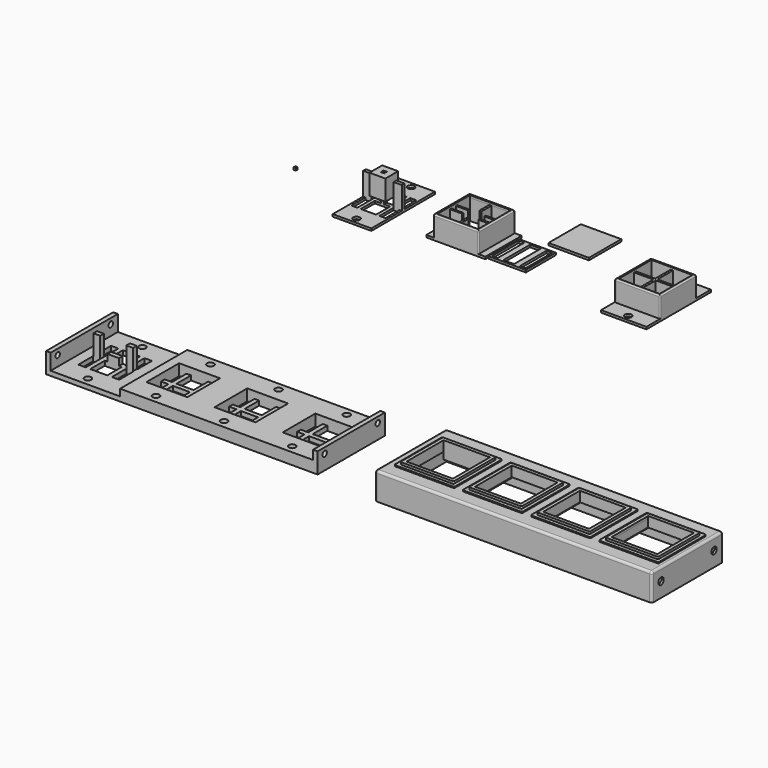
from build123d import *

# Parameters (mm, degrees)
F0_W          = 20
F0_H          = 20
F1_DEPTH      = 10
F2_T          = -1
F4_DEPTH      = 9
F5_W          = 20
F5_H          = 8
F5_R          = 1.5
F6_DEPTH      = 1
F7_W          = 20
F7_H          = 20
F8_DEPTH      = 10
F9_W          = 3
F9_H          = 20
F9_W_2        = 20
F10_DEPTH     = 0.95
F11_T         = 1
F11_T3_DEPTH  = 22
F12_W         = 8.5
F12_H         = 0.8
F13_DEPTH     = 9
F15_DEPTH     = 9
F16_W         = 17
F16_H         = 8
F16_R         = 1.5
F16_H_2       = 19
F17_DEPTH     = 1
F18_W         = 1.5
F18_H         = 1.5
F19_DEPTH     = 3
F20_W         = 7
F20_H         = 7
F20_W_2       = 1.5
F20_H_2       = 1.5
F21_DEPTH     = 9
F22_W         = 1
F22_H         = 1
F23_DEPTH     = 1
F25_DEPTH     = 10
F26_W         = 0.9
F26_H         = 14.7
F26_W_2       = 2.5
F26_H_2       = 0.8
F26_H_3       = 6
F26_H_4       = 1.1
F27_DEPTH     = 1
F28_W         = 117
F28_H         = 37
F28_R         = 1.5
F29_DEPTH     = 1
F30_W         = 122
F30_H         = 39.2
F30_W_2       = 20.4
F30_H_2       = 20.4
F30_W_3       = 20.2
F30_H_3       = 20.2
F31_DEPTH     = 11
F32_W         = 120
F32_H         = 37.2
F33_DEPTH     = 8
F34_W         = 4
F34_H         = 18
F35_DEPTH     = 3
F37_W         = 3
F37_H         = 2
F38_DEPTH     = 9
F39_W         = 5
F39_H         = 2
F40_DEPTH     = 3
F41_R         = 1
F42_R         = 0.5
F42_2_R       = 0.5
F36_R         = 1.5
F43_DEPTH     = 3
F44_DEPTH     = 2
F45_W         = 2
F45_H         = 37
F46_DEPTH     = 7
F47_W         = 20.4
F47_H         = 8.4
F48_DEPTH     = 3
F49_R         = 1.5
F50_DEPTH     = 3
F52_R         = 1.5
F53_DEPTH     = 2
F54_W         = 3
F54_H         = 37.2
F55_DEPTH     = 1
F56_DEPTH     = 1
F57_W         = 2
F57_H         = 37
F58_DEPTH     = 4
F51_R         = 1.2
F59_DEPTH     = 269.2358512024
F60_DEPTH     = 3
F61_DEPTH     = 5
F44_FACE2_W   = 119
F44_FACE2_H   = 37
F44_FACE2_R   = 1.5
F44_FACE2_W_2 = 3.25
F44_FACE2_H_2 = 8
F44_FACE2_W_3 = 7.5
F62_DEPTH     = 1
F63_DEPTH     = 1
F64_DEPTH     = 2
F65_DEPTH     = 0.05
F66_W         = 20.4
F66_H         = 3
F66_W_2       = 20.2
F66_H_2       = 3.1
F67_DEPTH     = 0.5
F68_W         = 20.4
F68_H         = 1.5
F68_W_2       = 20.2
F69_DEPTH     = 1
F70_R         = 0.5
F71_W         = 18
F71_H         = 17.9999990673
F72_DEPTH     = 1
F73_W         = 17.8
F73_H         = 17.8
F74_DEPTH     = 1
F75_W         = 18
F75_H         = 18
F76_DEPTH     = 1


# Not quite as in the source:
# - a shell that OpenCascade refuses in one call is made with other operations: the cavity is built on its own and cut out
# - a feature names something its author has since deleted; it is built from what else it names


with BuildPart() as f1:
    # F0 (on Top) → F1 (new body)
    with BuildSketch(Plane.XY):
        Rectangle(F0_W, F0_H)
    extrude(amount=F1_DEPTH)

    # F2
    f2_openings = [f1.faces().sort_by_distance(p)[0] for p in [
        (0, 0, 0),
    ]]
    offset(amount=F2_T, openings=f2_openings)

    # F3 (on Top) → F4 (join)
    with BuildSketch(Plane.XY):
        Polygon((-0.5, -9), (0.5, -9), (0.5, -0.5), (9, -0.5), (9, 0.5), (0.5, 0.5), (0.5, 9), (-0.5, 9), (-0.5, 0.5), (-9, 0.5), (-9, -0.5), (-0.5, -0.5), align=None)
    extrude(amount=F4_DEPTH)

    # F5 (on Top) → F6 (join)
    with BuildSketch(Plane.XY):
        with Locations((0, -13.5)):
            Rectangle(F5_W, F5_H)
        with Locations((0, -15)):
            Circle(F5_R, mode=Mode.SUBTRACT)
        with Locations((0, 14)):
            Rectangle(F5_W, F5_H)
        with Locations((0, 15)):
            Circle(F5_R, mode=Mode.SUBTRACT)
    extrude(amount=F6_DEPTH)

    # F42
    f42_edges = [f1.edges().sort_by_distance(p)[0] for p in [
        (-10, -10, 5.5),
        (0, -10, 10),
        (10, -10, 5.5),
        (-10, 0, 10),
        (-10, 10, 5.5),
        (0, 10, 10),
        (10, 10, 5.5),
        (10, 0, 10),
    ]]
    fillet(f42_edges, radius=F42_R)

    # F75 (on face) → F76 (cut)
    with BuildSketch(Plane.XY.offset(10)):
        Rectangle(F75_W, F75_H)
    extrude(amount=-F76_DEPTH, mode=Mode.SUBTRACT)


with BuildPart() as f8:
    # F7 (on Top) → F8 (new body)
    with BuildSketch(Plane.XY):
        with Locations((-78.8846665621, -1.3073290847)):
            Rectangle(F7_W, F7_H)
    extrude(amount=F8_DEPTH)

    # F9 (on face) → F10 (join)
    with BuildSketch(Plane(origin=(0, 0, 0), x_dir=(1, 0, 0), z_dir=(0, 0, -1))):
        with Locations((-90.3846665621, 1.3073290847)):
            Rectangle(F9_W, F9_H)
        with Locations((-78.8846665621, 1.3073290847)):
            Rectangle(F9_W_2, F9_H)
        with Locations((-67.3846665621, 1.3073290847)):
            Rectangle(F9_W, F9_H)
    extrude(amount=-F10_DEPTH)

    # F11: shell of thickness 1, made by hand


with BuildPart() as f11_core1:
    # F11_t2: copy of F8
    add(f8.part)

    # the walls: a layer under each face that stays
    f11_faces = [f11_core1.faces().sort_by_distance(p)[0] for p in [
        (-78.8846665621, 8.6926709153, 5),
        (-91.8846665621, -1.3073290847, 0.475),
        (-78.8846665621, -11.3073290847, 5),
        (-90.3846665621, -1.3073290847, 0.95),
        (-88.8846665621, -1.3073290847, 5.475),
        (-78.8846665621, -1.3073290847, 10),
        (-68.8846665621, -1.3073290847, 5.475),
        (-67.3846665621, -1.3073290847, 0.95),
        (-65.8846665621, -1.3073290847, 0.475),
    ]]
    thicken(f11_faces, amount=-F11_T, mode=Mode.SUBTRACT)

    # F11_s4 → F11_t3 (cut)
    with BuildSketch(Plane.XZ.offset(-9.6926709153)):
        Polygon((-88.8946665621, 0.96), (-88.8846665621, -0.05), (-87.8846665621, -0.05), (-87.8846665621, 0.95), align=None)
        Polygon((-68.8746665621, 0.96), (-69.8846665621, 0.95), (-69.8846665621, -0.05), (-68.8846665621, -0.05), align=None)
    extrude(amount=F11_T3_DEPTH, mode=Mode.SUBTRACT)


with BuildPart() as f8_1:
    add(f8.part)

    # what is left inside the walls is the cavity
    f11_cavity = [f11_core1.part.solids().sort_by_distance(p)[0] for p in [
        (-78.884667, -4.307329, 0.01),
    ]]
    add(f11_cavity, mode=Mode.SUBTRACT)

    # F12 (on Top) → F13 (join)
    with BuildSketch(Plane.XY):
        Polygon((-78.3846665621, 7.6926709153), (-79.3846665621, 7.6926709153), (-79.3846665621, 0.6926709153), (-79.3846665621, -0.1073290847), (-79.3846665621, -2.5073290847), (-79.3846665621, -3.3073290847), (-79.3846665621, -10.3073290847), (-78.3846665621, -10.3073290847), (-78.3846665621, -3.3073290847), (-78.3846665621, -2.5073290847), (-78.3846665621, -0.1073290847), (-78.3846665621, 0.6926709153), align=None)
        with Locations((-83.6346665621, -2.9073290847)):
            Rectangle(F12_W, F12_H)
        with Locations((-83.6346665621, 0.2926709153)):
            Rectangle(F12_W, F12_H)
        with Locations((-74.1346665621, 0.2926709153)):
            Rectangle(F12_W, F12_H)
        with Locations((-74.1346665621, -2.9073290847)):
            Rectangle(F12_W, F12_H)
    extrude(amount=F13_DEPTH)

    # F14 (on face) → F15 (cut)
    with BuildSketch(Plane(origin=(0, 0, 0), x_dir=(1, 0, 0), z_dir=(0, 0, -1))):
        Polygon((-79.3846665621, -2.2926709153), (-78.3846665621, -2.2926709153), (-78.3846665621, -0.6926709153), (-75.2846665621, -0.6926709153), (-75.2846665621, 0.1073290847), (-78.3846665621, 0.1073290847), (-78.3846665621, 2.5073290847), (-75.2846665621, 2.5073290847), (-75.2846665621, 3.3073290847), (-78.3846665621, 3.3073290847), (-78.3846665621, 4.9073290847), (-79.3846665621, 4.9073290847), (-79.3846665621, 3.3073290847), (-82.4846665621, 3.3073290847), (-82.4846665621, 2.5073290847), (-79.3846665621, 2.5073290847), (-79.3846665621, 0.1073290847), (-82.4846665621, 0.1073290847), (-82.4846665621, -0.6926709153), (-79.3846665621, -0.6926709153), align=None)
    extrude(amount=-F15_DEPTH, mode=Mode.SUBTRACT)

    # F42#2
    f42_2_edges = [f8_1.edges().sort_by_distance(p)[0] for p in [
        (-68.884667, -11.307329, 5.475),
        (-78.884667, -11.307329, 10),
        (-68.884667, -1.307329, 10),
        (-68.884667, 8.692671, 5.475),
        (-78.884667, 8.692671, 10),
        (-88.884667, 8.692671, 5.475),
        (-88.884667, -1.307329, 10),
        (-88.884667, -11.307329, 5.475),
    ]]
    fillet(f42_2_edges, radius=F42_2_R)

    # F65 (add): faces of the model
    f65_faces = [f8_1.faces().sort_by_distance(p)[0] for p in [
        (-90.3817894545, -1.3073290847, 0.95),
        (-67.3875436696, -1.3073290847, 0.95),
    ]]
    extrude(f65_faces, amount=F65_DEPTH)

    # F71 (on face) → F72 (cut)
    with BuildSketch(Plane.XY.offset(10)):
        with Locations((-78.8846665621, -1.3073295511)):
            Rectangle(F71_W, F71_H)
    extrude(amount=-F72_DEPTH, mode=Mode.SUBTRACT)


with BuildPart() as f17:
    # F16 (on Top) → F17 (new body)
    with BuildSketch(Plane.XY):
        with Locations((-118.1940851788, 11.6607970074)):
            Rectangle(F16_W, F16_H)
        with Locations((-118.1940851788, 13.1607970074)):
            Circle(F16_R, mode=Mode.SUBTRACT)
        with Locations((-118.1940851788, -15.3392029926)):
            Rectangle(F16_W, F16_H)
        with Locations((-118.1940851788, -16.8392029926)):
            Circle(F16_R, mode=Mode.SUBTRACT)
        with Locations((-118.1940851788, -1.8392029926)):
            Rectangle(F16_W, F16_H_2)
        Polygon((-125.6940851788, -1.0892029926), (-125.6940851788, 6.6607970074), (-123.0690851788, 6.6607970074), (-121.5690851788, 6.6607970074), (-114.8190851788, 6.6607970074), (-113.3190851788, 6.6607970074), (-110.6940851788, 6.6607970074), (-110.6940851788, -1.0892029926), (-110.6940851788, -2.5892029926), (-110.6940851788, -10.3392029926), (-113.3190851788, -10.3392029926), (-114.8190851788, -10.3392029926), (-121.5690851788, -10.3392029926), (-123.0690851788, -10.3392029926), (-125.6940851788, -10.3392029926), (-125.6940851788, -2.5892029926), align=None, mode=Mode.SUBTRACT)
        Polygon((-121.5690851788, 6.6607970074), (-123.0690851788, 6.6607970074), (-123.0690851788, -1.0892029926), (-125.6940851788, -1.0892029926), (-125.6940851788, -2.5892029926), (-123.0690851788, -2.5892029926), (-123.0690851788, -10.3392029926), (-121.5690851788, -10.3392029926), (-121.5690851788, -2.5892029926), (-114.8190851788, -2.5892029926), (-114.8190851788, -10.3392029926), (-113.3190851788, -10.3392029926), (-113.3190851788, -2.5892029926), (-110.6940851788, -2.5892029926), (-110.6940851788, -1.0892029926), (-113.3190851788, -1.0892029926), (-113.3190851788, 6.6607970074), (-114.8190851788, 6.6607970074), (-114.8190851788, -1.0892029926), (-121.5690851788, -1.0892029926), align=None)
    extrude(amount=F17_DEPTH)

    # F18 (on face) → F19 (join)
    with BuildSketch(Plane.XY.offset(1)):
        with Locations((-118.1940851788, -1.8392029926)):
            Rectangle(F18_W, F18_H)
    extrude(amount=F19_DEPTH)

    # F24 (on face) → F25 (join)
    with BuildSketch(Plane.XY.offset(1)):
        Polygon((-109.6940851788, -2.5892029926), (-109.6940851788, -1.0892029926), (-110.6940851788, -1.0892029926), (-113.3190851788, -1.0892029926), (-113.3190851788, -2.5892029926), (-110.6940851788, -2.5892029926), align=None)
        Polygon((-125.6940851788, -1.0892029926), (-126.6940851788, -1.0892029926), (-126.6940851788, -2.5892029926), (-125.6940851788, -2.5892029926), (-123.0690851788, -2.5892029926), (-123.0690851788, -1.0892029926), align=None)
    extrude(amount=F25_DEPTH)


with BuildPart() as f21:
    # F20 (on face) → F21 (new body)
    with BuildSketch(Plane.XY.offset(4)):
        with Locations((-118.1940851788, -1.8392029926)):
            Rectangle(F20_W, F20_H)
        with Locations((-118.1940851788, -1.8392029926)):
            Rectangle(F20_W_2, F20_H_2, mode=Mode.SUBTRACT)
    extrude(amount=F21_DEPTH)


with BuildPart() as f23:
    # F22 (on Top) → F23 (new body)
    with BuildSketch(Plane.XY):
        with Locations((-158.5527062416, 0)):
            Rectangle(F22_W, F22_H)
    extrude(amount=F23_DEPTH)


with BuildPart() as f27:
    # F26 (on Top) → F27 (new body)
    with BuildSketch(Plane.XY):
        Polygon((-64.4713718057, -9.4157041669), (-65.3713718057, -9.4157041669), (-65.3713718057, -10.3157041669), (-54.7713718057, -10.3157041669), (-52.2713718057, -10.3157041669), (-48.8713718057, -10.3157041669), (-48.8713718057, -9.4157041669), (-49.7713718057, -9.4157041669), (-52.2713718057, -9.4157041669), (-54.7713718057, -9.4157041669), (-59.4713718057, -9.4157041669), (-61.9713718057, -9.4157041669), align=None)
        with Locations((-64.9213718057, -2.0657041669)):
            Rectangle(F26_W, F26_H)
        Polygon((-48.8713718057, 6.1842958331), (-65.3713718057, 6.1842958331), (-65.3713718057, 5.2842958331), (-64.4713718057, 5.2842958331), (-61.9713718057, 5.2842958331), (-59.4713718057, 5.2842958331), (-54.7713718057, 5.2842958331), (-52.2713718057, 5.2842958331), (-49.7713718057, 5.2842958331), (-48.8713718057, 5.2842958331), align=None)
        with Locations((-49.3213718057, -2.0657041669)):
            Rectangle(F26_W, F26_H)
        with Locations((-53.5213718057, 4.8842958331)):
            Rectangle(F26_W_2, F26_H_2)
        with Locations((-53.5213718057, 1.4842958331)):
            Rectangle(F26_W_2, F26_H_3)
        with Locations((-53.5213718057, -2.0657041669)):
            Rectangle(F26_W_2, F26_H_4)
        with Locations((-53.5213718057, -5.6157041669)):
            Rectangle(F26_W_2, F26_H_3)
        with Locations((-53.5213718057, -9.0157041669)):
            Rectangle(F26_W_2, F26_H_2)
        with Locations((-60.7213718057, 4.8842958331)):
            Rectangle(F26_W_2, F26_H_2)
        with Locations((-60.7213718057, 1.4842958331)):
            Rectangle(F26_W_2, F26_H_3)
        with Locations((-60.7213718057, -2.0657041669)):
            Rectangle(F26_W_2, F26_H_4)
        with Locations((-60.7213718057, -5.6157041669)):
            Rectangle(F26_W_2, F26_H_3)
        with Locations((-60.7213718057, -9.0157041669)):
            Rectangle(F26_W_2, F26_H_2)
    extrude(amount=F27_DEPTH)


with BuildPart() as f29:
    # F28 (on Top) → F29 (new body)
    with BuildSketch(Plane.XY):
        with Locations((-71.0754835367, -152.5580135584)):
            Rectangle(F28_W, F28_H)
        with Locations((-115.9754835367, -167.5580135584)):
            Circle(F28_R, mode=Mode.SUBTRACT)
        with Locations((-85.9754835367, -167.5580135584)):
            Circle(F28_R, mode=Mode.SUBTRACT)
        Polygon((-124.9754835367, -151.5580135584), (-124.9754835367, -143.5580135584), (-121.7254835367, -143.5580135584), (-119.7254835367, -143.5580135584), (-112.2254835367, -143.5580135584), (-110.2254835367, -143.5580135584), (-106.9754835367, -143.5580135584), (-106.9754835367, -151.5580135584), (-106.9754835367, -153.5580135584), (-106.9754835367, -161.5580135584), (-110.2254835367, -161.5580135584), (-112.2254835367, -161.5580135584), (-119.7254835367, -161.5580135584), (-121.7254835367, -161.5580135584), (-124.9754835367, -161.5580135584), (-124.9754835367, -153.5580135584), align=None, mode=Mode.SUBTRACT)
        Polygon((-94.9754835367, -151.5580135584), (-94.9754835367, -143.5580135584), (-91.7254835367, -143.5580135584), (-89.7254835367, -143.5580135584), (-82.2254835367, -143.5580135584), (-80.2254835367, -143.5580135584), (-76.9754835367, -143.5580135584), (-76.9754835367, -151.5580135584), (-76.9754835367, -153.5580135584), (-76.9754835367, -161.5580135584), (-80.2254835367, -161.5580135584), (-82.2254835367, -161.5580135584), (-89.7254835367, -161.5580135584), (-91.7254835367, -161.5580135584), (-94.9754835367, -161.5580135584), (-94.9754835367, -153.5580135584), align=None, mode=Mode.SUBTRACT)
        with Locations((-55.9754835367, -167.5580135584)):
            Circle(F28_R, mode=Mode.SUBTRACT)
        with Locations((-25.9754835367, -167.5580135584)):
            Circle(F28_R, mode=Mode.SUBTRACT)
        Polygon((-64.9754835367, -151.5580135584), (-64.9754835367, -143.5580135584), (-61.7254835367, -143.5580135584), (-59.7254835367, -143.5580135584), (-52.2254835367, -143.5580135584), (-50.2254835367, -143.5580135584), (-46.9754835367, -143.5580135584), (-46.9754835367, -151.5580135584), (-46.9754835367, -153.5580135584), (-46.9754835367, -161.5580135584), (-47.9754835367, -161.5580135584), (-50.2254835367, -161.5580135584), (-52.2254835367, -161.5580135584), (-59.7254835367, -161.5580135584), (-61.7254835367, -161.5580135584), (-64.9754835367, -161.5580135584), (-64.9754835367, -153.5580135584), align=None, mode=Mode.SUBTRACT)
        Polygon((-34.9754835367, -151.5580135584), (-34.9754835367, -143.5580135584), (-31.7254835367, -143.5580135584), (-29.7254835367, -143.5580135584), (-22.2254835367, -143.5580135584), (-20.2254835367, -143.5580135584), (-16.9754835367, -143.5580135584), (-16.9754835367, -151.5580135584), (-16.9754835367, -153.5580135584), (-16.9754835367, -161.5580135584), (-17.9754835367, -161.5580135584), (-20.2254835367, -161.5580135584), (-22.2254835367, -161.5580135584), (-29.7254835367, -161.5580135584), (-31.7254835367, -161.5580135584), (-34.9754835367, -161.5580135584), (-34.9754835367, -153.5580135584), align=None, mode=Mode.SUBTRACT)
        with Locations((-115.9754835367, -137.5580135584)):
            Circle(F28_R, mode=Mode.SUBTRACT)
        with Locations((-85.9754835367, -137.5580135584)):
            Circle(F28_R, mode=Mode.SUBTRACT)
        with Locations((-55.9754835367, -137.5580135584)):
            Circle(F28_R, mode=Mode.SUBTRACT)
        with Locations((-25.9754835367, -137.5580135584)):
            Circle(F28_R, mode=Mode.SUBTRACT)
        Polygon((-119.7254835367, -143.5580135584), (-121.7254835367, -143.5580135584), (-121.7254835367, -151.5580135584), (-124.9754835367, -151.5580135584), (-124.9754835367, -153.5580135584), (-121.7254835367, -153.5580135584), (-121.7254835367, -161.5580135584), (-119.7254835367, -161.5580135584), (-119.7254835367, -153.5580135584), (-112.2254835367, -153.5580135584), (-112.2254835367, -161.5580135584), (-110.2254835367, -161.5580135584), (-110.2254835367, -153.5580135584), (-106.9754835367, -153.5580135584), (-106.9754835367, -151.5580135584), (-110.2254835367, -151.5580135584), (-110.2254835367, -143.5580135584), (-112.2254835367, -143.5580135584), (-112.2254835367, -151.5580135584), (-119.7254835367, -151.5580135584), align=None)
        Polygon((-89.7254835367, -143.5580135584), (-91.7254835367, -143.5580135584), (-91.7254835367, -151.5580135584), (-94.9754835367, -151.5580135584), (-94.9754835367, -153.5580135584), (-91.7254835367, -153.5580135584), (-91.7254835367, -161.5580135584), (-89.7254835367, -161.5580135584), (-89.7254835367, -153.5580135584), (-82.2254835367, -153.5580135584), (-82.2254835367, -161.5580135584), (-80.2254835367, -161.5580135584), (-80.2254835367, -153.5580135584), (-76.9754835367, -153.5580135584), (-76.9754835367, -151.5580135584), (-80.2254835367, -151.5580135584), (-80.2254835367, -143.5580135584), (-82.2254835367, -143.5580135584), (-82.2254835367, -151.5580135584), (-89.7254835367, -151.5580135584), align=None)
        Polygon((-59.7254835367, -143.5580135584), (-61.7254835367, -143.5580135584), (-61.7254835367, -151.5580135584), (-64.9754835367, -151.5580135584), (-64.9754835367, -153.5580135584), (-61.7254835367, -153.5580135584), (-61.7254835367, -161.5580135584), (-59.7254835367, -161.5580135584), (-59.7254835367, -153.5580135584), (-52.2254835367, -153.5580135584), (-52.2254835367, -161.5580135584), (-50.2254835367, -161.5580135584), (-50.2254835367, -153.5580135584), (-46.9754835367, -153.5580135584), (-46.9754835367, -151.5580135584), (-50.2254835367, -151.5580135584), (-50.2254835367, -143.5580135584), (-52.2254835367, -143.5580135584), (-52.2254835367, -151.5580135584), (-59.7254835367, -151.5580135584), align=None)
        Polygon((-29.7254835367, -143.5580135584), (-31.7254835367, -143.5580135584), (-31.7254835367, -151.5580135584), (-34.9754835367, -151.5580135584), (-34.9754835367, -153.5580135584), (-31.7254835367, -153.5580135584), (-31.7254835367, -161.5580135584), (-29.7254835367, -161.5580135584), (-29.7254835367, -153.5580135584), (-22.2254835367, -153.5580135584), (-22.2254835367, -161.5580135584), (-20.2254835367, -161.5580135584), (-20.2254835367, -153.5580135584), (-16.9754835367, -153.5580135584), (-16.9754835367, -151.5580135584), (-20.2254835367, -151.5580135584), (-20.2254835367, -143.5580135584), (-22.2254835367, -143.5580135584), (-22.2254835367, -151.5580135584), (-29.7254835367, -151.5580135584), align=None)
    extrude(amount=F29_DEPTH)

    # F34 (on face) → F35 (join)
    with BuildSketch(Plane.XY.offset(1)):
        with Locations((-96.9754835367, -152.5580135584)):
            Rectangle(F34_W, F34_H)
        with Locations((-74.9754835367, -152.5580135584)):
            Rectangle(F34_W, F34_H)
        with Locations((-66.9754835367, -152.5580135584)):
            Rectangle(F34_W, F34_H)
        with Locations((-44.9754835367, -152.5580135584)):
            Rectangle(F34_W, F34_H)
        with Locations((-36.9754835367, -152.5580135584)):
            Rectangle(F34_W, F34_H)
        with Locations((-14.9754835367, -152.5580135584)):
            Rectangle(F34_W, F34_H)
    extrude(amount=F35_DEPTH)

    # F37 (on face) → F38 (join)
    with BuildSketch(Plane.XY.offset(1)):
        with Locations((-123.2254835367, -152.5580135584)):
            Rectangle(F37_W, F37_H)
        with Locations((-108.7254835367, -152.5580135584)):
            Rectangle(F37_W, F37_H)
    extrude(amount=F38_DEPTH)

    # F39 (on face) → F40 (join)
    with BuildSketch(Plane.XY.offset(1)):
        with Locations((-115.9754835367, -152.5580135584)):
            Rectangle(F39_W, F39_H)
    extrude(amount=F40_DEPTH)

    # F36 (on face) → F43 (join)
    with BuildSketch(Plane.XY.offset(1)):
        Polygon((-98.9754835367, -134.0580135584), (-98.9754835367, -143.5580135584), (-94.9754835367, -143.5580135584), (-91.7254835367, -143.5580135584), (-89.7254835367, -143.5580135584), (-82.2254835367, -143.5580135584), (-80.2254835367, -143.5580135584), (-76.9754835367, -143.5580135584), (-72.9754835367, -143.5580135584), (-72.9754835367, -134.0580135584), align=None)
        with Locations((-85.9754835367, -137.5580135584)):
            Circle(F36_R, mode=Mode.SUBTRACT)
        Polygon((-94.9754835367, -161.5580135584), (-98.9754835367, -161.5580135584), (-98.9754835367, -171.0580135584), (-72.9754835367, -171.0580135584), (-72.9754835367, -161.5580135584), (-76.9754835367, -161.5580135584), (-80.2254835367, -161.5580135584), (-82.2254835367, -161.5580135584), (-89.7254835367, -161.5580135584), (-91.7254835367, -161.5580135584), align=None)
        with Locations((-85.9754835367, -167.5580135584)):
            Circle(F36_R, mode=Mode.SUBTRACT)
        Polygon((-68.9754835367, -161.5580135584), (-68.9754835367, -171.0580135584), (-42.9754835367, -171.0580135584), (-42.9754835367, -161.5580135584), (-46.9754835367, -161.5580135584), (-50.2254835367, -161.5580135584), (-52.2254835367, -161.5580135584), (-59.7254835367, -161.5580135584), (-61.7254835367, -161.5580135584), (-64.9754835367, -161.5580135584), align=None)
        with Locations((-55.9754835367, -167.5580135584)):
            Circle(F36_R, mode=Mode.SUBTRACT)
        Polygon((-42.9754835367, -134.0580135584), (-68.9754835367, -134.0580135584), (-68.9754835367, -143.5580135584), (-64.9754835367, -143.5580135584), (-61.7254835367, -143.5580135584), (-59.7254835367, -143.5580135584), (-52.2254835367, -143.5580135584), (-50.2254835367, -143.5580135584), (-46.9754835367, -143.5580135584), (-42.9754835367, -143.5580135584), align=None)
        with Locations((-55.9754835367, -137.5580135584)):
            Circle(F36_R, mode=Mode.SUBTRACT)
        Polygon((-12.9754835367, -134.0580135584), (-38.9754835367, -134.0580135584), (-38.9754835367, -143.5580135584), (-34.9754835367, -143.5580135584), (-31.7254835367, -143.5580135584), (-29.7254835367, -143.5580135584), (-22.2254835367, -143.5580135584), (-20.2254835367, -143.5580135584), (-16.9754835367, -143.5580135584), (-12.9754835367, -143.5580135584), align=None)
        with Locations((-25.9754835367, -137.5580135584)):
            Circle(F36_R, mode=Mode.SUBTRACT)
        Polygon((-38.9754835367, -161.5580135584), (-38.9754835367, -171.0580135584), (-12.9754835367, -171.0580135584), (-12.9754835367, -161.5580135584), (-16.9754835367, -161.5580135584), (-20.2254835367, -161.5580135584), (-22.2254835367, -161.5580135584), (-29.7254835367, -161.5580135584), (-31.7254835367, -161.5580135584), (-34.9754835367, -161.5580135584), align=None)
        with Locations((-25.9754835367, -167.5580135584)):
            Circle(F36_R, mode=Mode.SUBTRACT)
    extrude(amount=F43_DEPTH)

    # F44 (add): a face of the model
    f44_faces = [f29.faces().sort_by_distance(p)[0] for p in [
        (-129.5754835367, -152.5580135584, 0.5),
    ]]
    extrude(f44_faces, amount=F44_DEPTH)

    # F45 (on face) → F46 (join)
    with BuildSketch(Plane.XY.offset(1)):
        with Locations((-130.5754835367, -152.5580135584)):
            Rectangle(F45_W, F45_H)
    extrude(amount=F46_DEPTH)

    # F56 (add): a face of the model
    f56_faces = [f29.faces().sort_by_distance(p)[0] for p in [
        (-12.9754835367, -152.5580135584, 2.5),
    ]]
    extrude(f56_faces, amount=F56_DEPTH)

    # F57 (on face) → F58 (join)
    with BuildSketch(Plane.XY.offset(4)):
        with Locations((-12.9754835367, -152.5580135584)):
            Rectangle(F57_W, F57_H)
    extrude(amount=F58_DEPTH)

    # F51 (on face) → F59 (cut, through all)
    with BuildSketch(Plane(origin=(-131.5754835367, 0, 0), x_dir=(0, -1, 0), z_dir=(-1, 0, 0))):
        with Locations((137.9580135584, 5.5)):
            Circle(F51_R)
        with Locations((167.1580135584, 5.5)):
            Circle(F51_R)
    extrude(amount=-F59_DEPTH, mode=Mode.SUBTRACT)

    # F61 (add): faces of the model
    f61_faces = [f29.faces().sort_by_distance(p)[0] for p in [
        (-72.9754835367, -152.5580135584, 2.5),
        (-42.9754835367, -152.5580135584, 2.5),
    ]]
    extrude(f61_faces, amount=F61_DEPTH)

    # F28 (on Top) + F44_face2 (on face) → F62 (join)
    with BuildSketch(Plane.XY):
        with Locations((-71.0754835367, -152.5580135584)):
            Rectangle(F28_W, F28_H)
        with Locations((-115.9754835367, -167.5580135584)):
            Circle(F28_R, mode=Mode.SUBTRACT)
        with Locations((-85.9754835367, -167.5580135584)):
            Circle(F28_R, mode=Mode.SUBTRACT)
        Polygon((-124.9754835367, -151.5580135584), (-124.9754835367, -143.5580135584), (-121.7254835367, -143.5580135584), (-119.7254835367, -143.5580135584), (-112.2254835367, -143.5580135584), (-110.2254835367, -143.5580135584), (-106.9754835367, -143.5580135584), (-106.9754835367, -151.5580135584), (-106.9754835367, -153.5580135584), (-106.9754835367, -161.5580135584), (-110.2254835367, -161.5580135584), (-112.2254835367, -161.5580135584), (-119.7254835367, -161.5580135584), (-121.7254835367, -161.5580135584), (-124.9754835367, -161.5580135584), (-124.9754835367, -153.5580135584), align=None, mode=Mode.SUBTRACT)
        Polygon((-94.9754835367, -151.5580135584), (-94.9754835367, -143.5580135584), (-91.7254835367, -143.5580135584), (-89.7254835367, -143.5580135584), (-82.2254835367, -143.5580135584), (-80.2254835367, -143.5580135584), (-76.9754835367, -143.5580135584), (-76.9754835367, -151.5580135584), (-76.9754835367, -153.5580135584), (-76.9754835367, -161.5580135584), (-80.2254835367, -161.5580135584), (-82.2254835367, -161.5580135584), (-89.7254835367, -161.5580135584), (-91.7254835367, -161.5580135584), (-94.9754835367, -161.5580135584), (-94.9754835367, -153.5580135584), align=None, mode=Mode.SUBTRACT)
        with Locations((-55.9754835367, -167.5580135584)):
            Circle(F28_R, mode=Mode.SUBTRACT)
        with Locations((-25.9754835367, -167.5580135584)):
            Circle(F28_R, mode=Mode.SUBTRACT)
        Polygon((-64.9754835367, -151.5580135584), (-64.9754835367, -143.5580135584), (-61.7254835367, -143.5580135584), (-59.7254835367, -143.5580135584), (-52.2254835367, -143.5580135584), (-50.2254835367, -143.5580135584), (-46.9754835367, -143.5580135584), (-46.9754835367, -151.5580135584), (-46.9754835367, -153.5580135584), (-46.9754835367, -161.5580135584), (-47.9754835367, -161.5580135584), (-50.2254835367, -161.5580135584), (-52.2254835367, -161.5580135584), (-59.7254835367, -161.5580135584), (-61.7254835367, -161.5580135584), (-64.9754835367, -161.5580135584), (-64.9754835367, -153.5580135584), align=None, mode=Mode.SUBTRACT)
        Polygon((-34.9754835367, -151.5580135584), (-34.9754835367, -143.5580135584), (-31.7254835367, -143.5580135584), (-29.7254835367, -143.5580135584), (-22.2254835367, -143.5580135584), (-20.2254835367, -143.5580135584), (-16.9754835367, -143.5580135584), (-16.9754835367, -151.5580135584), (-16.9754835367, -153.5580135584), (-16.9754835367, -161.5580135584), (-17.9754835367, -161.5580135584), (-20.2254835367, -161.5580135584), (-22.2254835367, -161.5580135584), (-29.7254835367, -161.5580135584), (-31.7254835367, -161.5580135584), (-34.9754835367, -161.5580135584), (-34.9754835367, -153.5580135584), align=None, mode=Mode.SUBTRACT)
        with Locations((-115.9754835367, -137.5580135584)):
            Circle(F28_R, mode=Mode.SUBTRACT)
        with Locations((-85.9754835367, -137.5580135584)):
            Circle(F28_R, mode=Mode.SUBTRACT)
        with Locations((-55.9754835367, -137.5580135584)):
            Circle(F28_R, mode=Mode.SUBTRACT)
        with Locations((-25.9754835367, -137.5580135584)):
            Circle(F28_R, mode=Mode.SUBTRACT)
    with BuildSketch(Plane(origin=(-72.3791549796, -152.5580135584, 0), x_dir=(1, 0, 0), z_dir=(0, 0, -1))):
        with Locations((0.3036714428, 0)):
            Rectangle(F44_FACE2_W, F44_FACE2_H)
        with Locations((-43.5963285572, 15)):
            Circle(F44_FACE2_R, mode=Mode.SUBTRACT)
        with Locations((-13.5963285572, 15)):
            Circle(F44_FACE2_R, mode=Mode.SUBTRACT)
        with Locations((-36.2213285572, 5)):
            Rectangle(F44_FACE2_W_2, F44_FACE2_H_2, mode=Mode.SUBTRACT)
        with Locations((-43.5963285572, 5)):
            Rectangle(F44_FACE2_W_3, F44_FACE2_H_2, mode=Mode.SUBTRACT)
        with Locations((-50.9713285572, 5)):
            Rectangle(F44_FACE2_W_2, F44_FACE2_H_2, mode=Mode.SUBTRACT)
        with Locations((-50.9713285572, -5)):
            Rectangle(F44_FACE2_W_2, F44_FACE2_H_2, mode=Mode.SUBTRACT)
        with Locations((-43.5963285572, -5)):
            Rectangle(F44_FACE2_W_3, F44_FACE2_H_2, mode=Mode.SUBTRACT)
        with Locations((-36.2213285572, -5)):
            Rectangle(F44_FACE2_W_2, F44_FACE2_H_2, mode=Mode.SUBTRACT)
        with Locations((-6.2213285572, 5)):
            Rectangle(F44_FACE2_W_2, F44_FACE2_H_2, mode=Mode.SUBTRACT)
        with Locations((-13.5963285572, 5)):
            Rectangle(F44_FACE2_W_3, F44_FACE2_H_2, mode=Mode.SUBTRACT)
        with Locations((-20.9713285572, 5)):
            Rectangle(F44_FACE2_W_2, F44_FACE2_H_2, mode=Mode.SUBTRACT)
        with Locations((-20.9713285572, -5)):
            Rectangle(F44_FACE2_W_2, F44_FACE2_H_2, mode=Mode.SUBTRACT)
        with Locations((-13.5963285572, -5)):
            Rectangle(F44_FACE2_W_3, F44_FACE2_H_2, mode=Mode.SUBTRACT)
        with Locations((-6.2213285572, -5)):
            Rectangle(F44_FACE2_W_2, F44_FACE2_H_2, mode=Mode.SUBTRACT)
        with Locations((16.4036714428, 15)):
            Circle(F44_FACE2_R, mode=Mode.SUBTRACT)
        with Locations((46.4036714428, 15)):
            Circle(F44_FACE2_R, mode=Mode.SUBTRACT)
        with Locations((23.7786714428, 5)):
            Rectangle(F44_FACE2_W_2, F44_FACE2_H_2, mode=Mode.SUBTRACT)
        with Locations((16.4036714428, 5)):
            Rectangle(F44_FACE2_W_3, F44_FACE2_H_2, mode=Mode.SUBTRACT)
        with Locations((9.0286714428, 5)):
            Rectangle(F44_FACE2_W_2, F44_FACE2_H_2, mode=Mode.SUBTRACT)
        with Locations((9.0286714428, -5)):
            Rectangle(F44_FACE2_W_2, F44_FACE2_H_2, mode=Mode.SUBTRACT)
        with Locations((16.4036714428, -5)):
            Rectangle(F44_FACE2_W_3, F44_FACE2_H_2, mode=Mode.SUBTRACT)
        with Locations((23.7786714428, -5)):
            Rectangle(F44_FACE2_W_2, F44_FACE2_H_2, mode=Mode.SUBTRACT)
        with Locations((53.7786714428, 5)):
            Rectangle(F44_FACE2_W_2, F44_FACE2_H_2, mode=Mode.SUBTRACT)
        with Locations((46.4036714428, 5)):
            Rectangle(F44_FACE2_W_3, F44_FACE2_H_2, mode=Mode.SUBTRACT)
        with Locations((39.0286714428, 5)):
            Rectangle(F44_FACE2_W_2, F44_FACE2_H_2, mode=Mode.SUBTRACT)
        with Locations((39.0286714428, -5)):
            Rectangle(F44_FACE2_W_2, F44_FACE2_H_2, mode=Mode.SUBTRACT)
        with Locations((46.4036714428, -5)):
            Rectangle(F44_FACE2_W_3, F44_FACE2_H_2, mode=Mode.SUBTRACT)
        with Locations((53.7786714428, -5)):
            Rectangle(F44_FACE2_W_2, F44_FACE2_H_2, mode=Mode.SUBTRACT)
        with Locations((-43.5963285572, -15)):
            Circle(F44_FACE2_R, mode=Mode.SUBTRACT)
        with Locations((-13.5963285572, -15)):
            Circle(F44_FACE2_R, mode=Mode.SUBTRACT)
        with Locations((16.4036714428, -15)):
            Circle(F44_FACE2_R, mode=Mode.SUBTRACT)
        with Locations((46.4036714428, -15)):
            Circle(F44_FACE2_R, mode=Mode.SUBTRACT)
    extrude(amount=-F62_DEPTH, dir=(0, 0, 1))

    # F64 (add): a face of the model
    f64_faces = [f29.faces().sort_by_distance(p)[0] for p in [
        (-12.2754835367, -152.5580135584, 1),
    ]]
    extrude(f64_faces, amount=F64_DEPTH)


with BuildPart() as f31:
    # F30 (on Top) → F31 (new body)
    with BuildSketch(Plane.XY):
        with Locations((76.6593676656, -154.4580135584)):
            Rectangle(F30_W, F30_H)
        with Locations((32.2593676656, -154.4580135584)):
            Rectangle(F30_W_2, F30_H_2, mode=Mode.SUBTRACT)
        with Locations((62.2593676656, -154.4580135584)):
            Rectangle(F30_W_3, F30_H_3, mode=Mode.SUBTRACT)
        with Locations((92.2593676656, -154.4580135584)):
            Rectangle(F30_W_3, F30_H_3, mode=Mode.SUBTRACT)
        with Locations((122.2593676656, -154.4580135584)):
            Rectangle(F30_W_3, F30_H_3, mode=Mode.SUBTRACT)
    extrude(amount=F31_DEPTH)

    # F32 (on face) → F33 (cut)
    with BuildSketch(Plane(origin=(0, 0, 0), x_dir=(1, 0, 0), z_dir=(0, 0, -1))):
        with Locations((76.6593676656, 154.4580135584)):
            Rectangle(F32_W, F32_H)
    extrude(amount=-F33_DEPTH, mode=Mode.SUBTRACT)

    # F41
    f41_edges = [f31.edges().sort_by_distance(p)[0] for p in [
        (15.659368, -134.858014, 5.5),
        (15.659368, -174.058014, 5.5),
        (137.659368, -174.058014, 5.5),
        (137.659368, -134.858014, 5.5),
        (76.659368, -174.058014, 11),
        (15.659368, -154.458014, 11),
        (76.659368, -134.858014, 11),
        (137.659368, -154.458014, 11),
    ]]
    fillet(f41_edges, radius=F41_R)

    # F47 (on face) → F48 (join)
    with BuildSketch(Plane(origin=(0, 0, 8), x_dir=(1, 0, 0), z_dir=(0, 0, -1))):
        with Locations((32.2593676656, 168.8580135584)):
            Rectangle(F47_W, F47_H)
        with Locations((32.2593676656, 140.0580135584)):
            Rectangle(F47_W, F47_H)
    extrude(amount=F48_DEPTH)

    # F49 (on face) → F50 (cut)
    with BuildSketch(Plane(origin=(15.6593676656, 0, 0), x_dir=(0, -1, 0), z_dir=(-1, 0, 0))):
        with Locations((139.8580135584, 5.5)):
            Circle(F49_R)
        with Locations((169.0580135584, 5.5)):
            Circle(F49_R)
    extrude(amount=-F50_DEPTH, mode=Mode.SUBTRACT)

    # F52 (on face) → F53 (cut)
    with BuildSketch(Plane.YZ.offset(137.6593676656)):
        with Locations((-169.0580135584, 5.5)):
            Circle(F52_R)
        with Locations((-139.8580135584, 5.5)):
            Circle(F52_R)
    extrude(amount=-F53_DEPTH, mode=Mode.SUBTRACT)

    # F54 (on face) → F55 (join)
    with BuildSketch(Plane(origin=(0, 0, 8), x_dir=(1, 0, 0), z_dir=(0, 0, -1))):
        with Locations((47.4593676656, 154.4580135584)):
            Rectangle(F54_W, F54_H)
        with Locations((77.3593676656, 154.4580135584)):
            Rectangle(F54_W, F54_H)
        with Locations((107.3593676656, 154.4580135584)):
            Rectangle(F54_W, F54_H)
    extrude(amount=F55_DEPTH)

    # F54 (on face) → F60 (join)
    with BuildSketch(Plane(origin=(0, 0, 8), x_dir=(1, 0, 0), z_dir=(0, 0, -1))):
        with Locations((47.4593676656, 154.4580135584)):
            Rectangle(F54_W, F54_H)
        with Locations((77.3593676656, 154.4580135584)):
            Rectangle(F54_W, F54_H)
        with Locations((107.3593676656, 154.4580135584)):
            Rectangle(F54_W, F54_H)
    extrude(amount=F60_DEPTH)

    # F63 (add): a face of the model
    f63_faces = [f31.faces().sort_by_distance(p)[0] for p in [
        (137.5312246206, -154.4580135584, 0),
    ]]
    extrude(f63_faces, amount=F63_DEPTH)

    # F66 (on face) → F67 (join)
    with BuildSketch(Plane.XY.offset(11)):
        with Locations((32.2593676656, -142.7580135584)):
            Rectangle(F66_W, F66_H)
        Polygon((22.0593676656, -164.6580135584), (22.0593676656, -144.2580135584), (22.0593676656, -141.2580135584), (19.0593676656, -141.2580135584), (19.0593676656, -167.6580135584), (22.0593676656, -167.6580135584), align=None)
        Polygon((42.4593676656, -141.2580135584), (42.4593676656, -144.2580135584), (42.4593676656, -164.6580135584), (42.4593676656, -167.6580135584), (45.4593676656, -167.6580135584), (45.4593676656, -141.2580135584), align=None)
        with Locations((32.2593676656, -166.1580135584)):
            Rectangle(F66_W, F66_H)
        with Locations((62.2593676656, -142.8080135584)):
            Rectangle(F66_W_2, F66_H_2)
        Polygon((52.1593676656, -164.5580135584), (52.1593676656, -144.3580135584), (52.1593676656, -141.2580135584), (49.1593676656, -141.2580135584), (49.1593676656, -167.6580135584), (52.1593676656, -167.6580135584), align=None)
        Polygon((72.3593676656, -141.2580135584), (72.3593676656, -144.3580135584), (72.3593676656, -164.5580135584), (72.3593676656, -167.6580135584), (75.3593676656, -167.6580135584), (75.3593676656, -141.2580135584), align=None)
        with Locations((62.2593676656, -166.1080135584)):
            Rectangle(F66_W_2, F66_H_2)
        with Locations((92.2593676656, -142.8080135584)):
            Rectangle(F66_W_2, F66_H_2)
        Polygon((82.1593676656, -164.5580135584), (82.1593676656, -144.3580135584), (82.1593676656, -141.2580135584), (79.1593676656, -141.2580135584), (79.1593676656, -167.6580135584), (82.1593676656, -167.6580135584), align=None)
        Polygon((102.3593676656, -141.2580135584), (102.3593676656, -144.3580135584), (102.3593676656, -164.5580135584), (102.3593676656, -167.6580135584), (105.3593676656, -167.6580135584), (105.3593676656, -141.2580135584), align=None)
        with Locations((92.2593676656, -166.1080135584)):
            Rectangle(F66_W_2, F66_H_2)
        with Locations((122.2593676656, -142.8080135584)):
            Rectangle(F66_W_2, F66_H_2)
        Polygon((112.1593676656, -164.5580135584), (112.1593676656, -144.3580135584), (112.1593676656, -141.2580135584), (109.1593676656, -141.2580135584), (109.1593676656, -167.6580135584), (112.1593676656, -167.6580135584), align=None)
        Polygon((132.3593676656, -141.2580135584), (132.3593676656, -144.3580135584), (132.3593676656, -164.5580135584), (132.3593676656, -167.6580135584), (135.3593676656, -167.6580135584), (135.3593676656, -141.2580135584), align=None)
        with Locations((122.2593676656, -166.1080135584)):
            Rectangle(F66_W_2, F66_H_2)
    extrude(amount=F67_DEPTH)

    # F68 (on face) → F69 (join)
    with BuildSketch(Plane.XY.offset(11.5)):
        with Locations((32.2593676656, -143.5080135584)):
            Rectangle(F68_W, F68_H)
        Polygon((22.0593676656, -164.6580135584), (22.0593676656, -144.2580135584), (22.0593676656, -142.7580135584), (20.5593676656, -142.7580135584), (20.5593676656, -166.1580135584), (22.0593676656, -166.1580135584), align=None)
        Polygon((42.4593676656, -142.7580135584), (42.4593676656, -144.2580135584), (42.4593676656, -164.6580135584), (42.4593676656, -166.1580135584), (43.9593676656, -166.1580135584), (43.9593676656, -142.7580135584), align=None)
        with Locations((32.2593676656, -165.4080135584)):
            Rectangle(F68_W, F68_H)
        Polygon((52.1593676656, -142.8580135584), (50.6593676656, -142.8580135584), (50.6593676656, -166.0580135584), (52.1593676656, -166.0580135584), (52.1593676656, -164.5580135584), (52.1593676656, -144.3580135584), align=None)
        with Locations((62.2593676656, -143.6080135584)):
            Rectangle(F68_W_2, F68_H)
        Polygon((73.8593676656, -142.8580135584), (72.3593676656, -142.8580135584), (72.3593676656, -144.3580135584), (72.3593676656, -164.5580135584), (72.3593676656, -166.0580135584), (73.8593676656, -166.0580135584), align=None)
        with Locations((62.2593676656, -165.3080135584)):
            Rectangle(F68_W_2, F68_H)
        Polygon((82.1593676656, -142.8580135584), (80.6593676656, -142.8580135584), (80.6593676656, -166.0580135584), (82.1593676656, -166.0580135584), (82.1593676656, -164.5580135584), (82.1593676656, -144.3580135584), align=None)
        with Locations((92.2593676656, -143.6080135584)):
            Rectangle(F68_W_2, F68_H)
        Polygon((103.8593676656, -142.8580135584), (102.3593676656, -142.8580135584), (102.3593676656, -144.3580135584), (102.3593676656, -164.5580135584), (102.3593676656, -166.0580135584), (103.8593676656, -166.0580135584), align=None)
        with Locations((92.2593676656, -165.3080135584)):
            Rectangle(F68_W_2, F68_H)
        Polygon((112.2593676656, -142.8580135584), (110.7593676656, -142.8580135584), (110.7593676656, -166.0580135584), (112.2593676656, -166.0580135584), (112.2593676656, -164.5580135584), (112.2593676656, -144.3580135584), align=None)
        with Locations((122.3593676656, -143.6080135584)):
            Rectangle(F68_W_2, F68_H)
        Polygon((133.9593676656, -142.8580135584), (132.4593676656, -142.8580135584), (132.4593676656, -144.3580135584), (132.4593676656, -164.5580135584), (132.4593676656, -166.0580135584), (133.9593676656, -166.0580135584), align=None)
        with Locations((122.3593676656, -165.3080135584)):
            Rectangle(F68_W_2, F68_H)
    extrude(amount=F69_DEPTH)

    # F70
    f70_edges = [f31.edges().sort_by_distance(p)[0] for p in [
        (19.059368, -141.258014, 11.25),
        (20.559368, -142.758014, 12),
        (19.059368, -167.658014, 11.25),
        (20.559368, -166.158014, 12),
        (43.959368, -166.158014, 12),
        (45.459368, -167.658014, 11.25),
        (43.959368, -142.758014, 12),
        (45.459368, -141.258014, 11.25),
        (49.159368, -141.258014, 11.25),
        (50.659368, -142.858014, 12),
        (50.659368, -166.058014, 12),
        (49.159368, -167.658014, 11.25),
        (73.859368, -166.058014, 12),
        (75.359368, -167.658014, 11.25),
        (73.859368, -142.858014, 12),
        (75.359368, -141.258014, 11.25),
        (79.159368, -141.258014, 11.25),
        (80.659368, -142.858014, 12),
        (79.159368, -167.658014, 11.25),
        (80.659368, -166.058014, 12),
        (103.859368, -166.058014, 12),
        (105.359368, -167.658014, 11.25),
        (103.859368, -142.858014, 12),
        (105.359368, -141.258014, 11.25),
        (109.159368, -141.258014, 11.25),
        (110.759368, -142.858014, 12),
        (109.159368, -167.658014, 11.25),
        (110.759368, -166.058014, 12),
        (133.959368, -166.058014, 12),
        (135.359368, -167.658014, 11.25),
        (133.959368, -142.858014, 12),
        (135.359368, -141.258014, 11.25),
    ]]
    fillet(f70_edges, radius=F70_R)


with BuildPart() as f74:
    # F73 (on Top) → F74 (new body)
    with BuildSketch(Plane.XY):
        with Locations((-46.4569205403, 19.1935256436)):
            Rectangle(F73_W, F73_H)
    extrude(amount=F74_DEPTH)


solid = Compound([f1.part, f8_1.part, f17.part, f21.part, f23.part, f27.part, f29.part, f31.part, f74.part])
